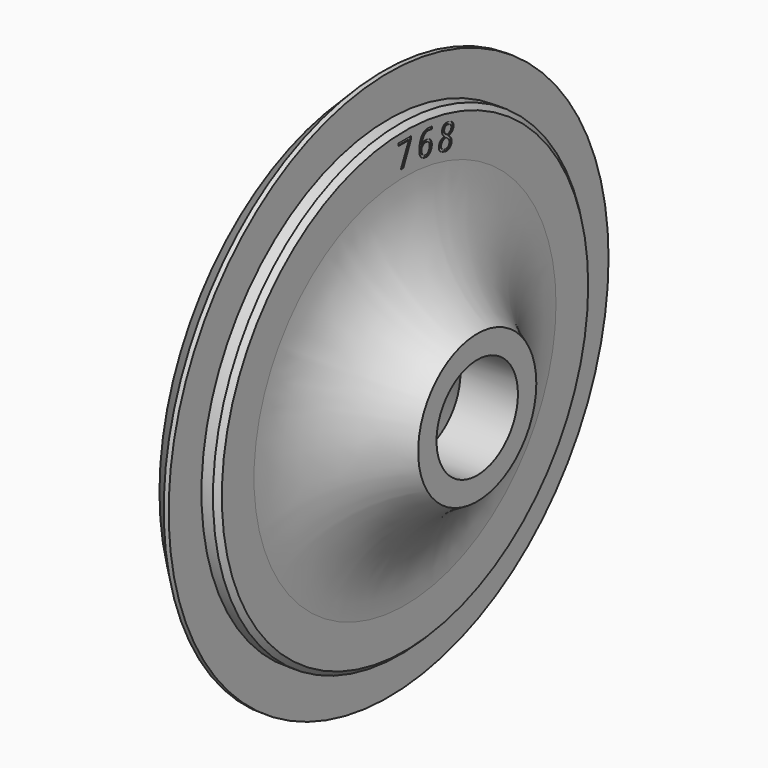
from build123d import *

# Parameters (mm, degrees)
F3_TEXT_SIZE = 2.0833333333
F4_DEPTH     = 0.05
F5_SIZE      = 0.3


# Not quite as in the source:
# - Text() gives the source's letters only with a copy of the font that has no kerning and outlines rounded to 1/6400 em; it was checked with that copy


with BuildPart() as f1:
    # F0 (on Top) → F1 (revolve)
    with BuildSketch(Plane.XY):
        with BuildLine():
            Line((-4.4, 11.5), (-4.4, 14.25))
            Line((-4.4, 14.25), (-5.4, 14.25))
            Line((-5.4, 14.25), (-5.4, 16.75))
            Line((-5.4, 16.75), (-5.7, 16.75))
            Line((-5.7, 16.75), (-7, 15.45))
            Line((-7, 15.45), (-7, 6))
            Line((-7, 6), (-6.4, 6))
            Line((-6.4, 6), (-3.5, 3.1))
            Line((-3.5, 3.1), (0, 3.1))
            Line((0, 3.1), (0, 4.5))
            ThreePointArc((0, 4.5), (-3.20864483, 7.3659946783), (-4.4, 11.5))
        make_face()
    revolve(axis=Axis((-3.5, 0, 0), (-1, 0, 0)))

    # F3 (on face) → F4 (cut)
    with BuildSketch(Plane.YZ.offset(-4.4)):
        with Locations((-0.6101888021, 12)):
            Text('7', F3_TEXT_SIZE, font='Open Sans', text_align=(TextAlign.LEFT, TextAlign.BOTTOM))
        with BuildLine():
            add(Edge.make_bspline(
                [(1.3911920227, 11.9124736168), (1.2492672408, 11.965505738), (1.168086207, 12.102022835)],
                knots=[0.2780169607, 0.2780169607, 0.2780169607, 1, 1, 1], degree=2))
            Line((1.3911920227, 11.9124736168), (1.5039988028, 11.9053764158))
            Line((1.5039988028, 11.9053764158), (1.6329910314, 11.8807698321))
            add(Edge.make_bspline(
                [(1.8658957751, 11.9728554781), (1.7668517571, 11.8921760098), (1.6329910314, 11.8807698321)],
                knots=[0, 0, 0, 0.6961452699, 0.6961452699, 0.6961452699], degree=2))
            add(Edge.make_bspline(
                [(2.0372600894, 12.3190162698), (2.0081707028, 12.0887500648), (1.8658957751, 11.9728554781)],
                knots=[0, 0, 0, 1, 1, 1], degree=2))
            add(Edge.make_bspline(
                [(1.9639386607, 12.6593399563), (2.063248784, 12.5247379706), (2.0372600894, 12.3190162698)],
                knots=[0, 0, 0, 1, 1, 1], degree=2))
            add(Edge.make_bspline(
                [(1.6656888708, 12.8190738665), (1.8646285374, 12.7939419421), (1.9639386607, 12.6593399563)],
                knots=[0, 0, 0, 1, 1, 1], degree=2))
            add(Edge.make_bspline(
                [(1.2923652787, 12.6897134657), (1.4254110915, 12.849428009), (1.6656888708, 12.8190738665)],
                knots=[0, 0, 0, 1, 1, 1], degree=2))
            Line((1.2923652787, 12.6897134657), (1.2804159806, 12.6912230132))
            add(Edge.make_bspline(
                [(1.4762395094, 13.1387963058), (1.332429483, 13.006854298), (1.2804159806, 12.6912230132)],
                knots=[0, 0, 0, 1, 1, 1], degree=2))
            add(Edge.make_bspline(
                [(1.8574207289, 13.2407513582), (1.6200495358, 13.2707383135), (1.4762395094, 13.1387963058)],
                knots=[0, 0, 0, 1, 1, 1], degree=2))
            add(Edge.make_bspline(
                [(2.0318631422, 13.1931217276), (1.9572135163, 13.2281445974), (1.8574207289, 13.2407513582)],
                knots=[0, 0, 0, 1, 1, 1], degree=2))
            Line((2.0318631422, 13.1931217276), (2.0501001068, 13.3374821676))
            add(Edge.make_bspline(
                [(1.8729447966, 13.3792204636), (1.9869475601, 13.3648185653), (2.0501001068, 13.3374821676)],
                knots=[0, 0, 0, 1, 1, 1], degree=2))
            add(Edge.make_bspline(
                [(1.3456378689, 13.2269867417), (1.5419169421, 13.4210390067), (1.8729447966, 13.3792204636)],
                knots=[0, 0, 0, 1, 1, 1], degree=2))
            add(Edge.make_bspline(
                [(1.0944031103, 12.5979154329), (1.1493587957, 13.0329344767), (1.3456378689, 13.2269867417)],
                knots=[0, 0, 0, 1, 1, 1], degree=2))
            add(Edge.make_bspline(
                [(1.168086207, 12.102022835), (1.0556444606, 12.2911091288), (1.0944031103, 12.5979154329)],
                knots=[0, 0, 0, 1, 1, 1], degree=2))
        make_face()
        with BuildLine():
            add(Edge.make_bspline(
                [(1.5255567916, 12.0266778564), (1.6689483695, 12.0085632875), (1.7594957026, 12.088994757)],
                knots=[0, 0, 0, 1, 1, 1], degree=2))
            add(Edge.make_bspline(
                [(1.3631201393, 12.100515938), (1.4306083143, 12.0386726385), (1.5255567916, 12.0266778564)],
                knots=[0, 0, 0, 1, 1, 1], degree=2))
            add(Edge.make_bspline(
                [(1.2666047187, 12.2572402731), (1.2956319644, 12.1623592375), (1.3631201393, 12.100515938)],
                knots=[0, 0, 0, 1, 1, 1], degree=2))
            add(Edge.make_bspline(
                [(1.2507146153, 12.456112498), (1.237577473, 12.3521213086), (1.2666047187, 12.2572402731)],
                knots=[0, 0, 0, 1, 1, 1], degree=2))
            add(Edge.make_bspline(
                [(1.3128222221, 12.5867280854), (1.259649504, 12.526839425), (1.2507146153, 12.456112498)],
                knots=[0, 0, 0, 1, 1, 1], degree=2))
            add(Edge.make_bspline(
                [(1.4464602893, 12.6745121437), (1.3659949402, 12.6466167459), (1.3128222221, 12.5867280854)],
                knots=[0, 0, 0, 1, 1, 1], degree=2))
            add(Edge.make_bspline(
                [(1.6176757137, 12.6909431409), (1.5269256385, 12.7024075415), (1.4464602893, 12.6745121437)],
                knots=[0, 0, 0, 1, 1, 1], degree=2))
            add(Edge.make_bspline(
                [(1.8270201595, 12.5793527447), (1.7639738776, 12.6724613848), (1.6176757137, 12.6909431409)],
                knots=[0, 0, 0, 1, 1, 1], degree=2))
            add(Edge.make_bspline(
                [(1.8715846852, 12.3399459407), (1.8900664413, 12.4862441047), (1.8270201595, 12.5793527447)],
                knots=[0, 0, 0, 1, 1, 1], degree=2))
            add(Edge.make_bspline(
                [(1.7594957026, 12.088994757), (1.8500430357, 12.1694262264), (1.8715846852, 12.3399459407)],
                knots=[0, 0, 0, 1, 1, 1], degree=2))
        make_face(mode=Mode.SUBTRACT)
        with BuildLine():
            Line((2.984278646, 11.6229979335), (3.1084826292, 11.582641613))
            add(Edge.make_bspline(
                [(3.3407163455, 11.6244062371), (3.239004536, 11.5744991717), (3.1084826292, 11.582641613)],
                knots=[0, 0, 0, 0.666283244, 0.666283244, 0.666283244], degree=2))
            add(Edge.make_bspline(
                [(3.5393535811, 11.8783969056), (3.4933718571, 11.6993099149), (3.3407163455, 11.6244062371)],
                knots=[0, 0, 0, 1, 1, 1], degree=2))
            add(Edge.make_bspline(
                [(3.5202228201, 12.1108345939), (3.5705207707, 11.9997850947), (3.5393535811, 11.8783969056)],
                knots=[0, 0, 0, 1, 1, 1], degree=2))
            add(Edge.make_bspline(
                [(3.3161551014, 12.3507625756), (3.4699248695, 12.2218840932), (3.5202228201, 12.1108345939)],
                knots=[0, 0, 0, 1, 1, 1], degree=2))
            add(Edge.make_bspline(
                [(3.568049378, 12.4561432869), (3.4796477929, 12.385410887), (3.3161551014, 12.3507625756)],
                knots=[0, 0, 0, 1, 1, 1], degree=2))
            add(Edge.make_bspline(
                [(3.683813327, 12.633445058), (3.6564509631, 12.5268756868), (3.568049378, 12.4561432869)],
                knots=[0, 0, 0, 1, 1, 1], degree=2))
            add(Edge.make_bspline(
                [(3.6335387466, 12.9160570829), (3.7252616415, 12.7948755848), (3.683813327, 12.633445058)],
                knots=[0, 0, 0, 1, 1, 1], degree=2))
            add(Edge.make_bspline(
                [(3.3447571031, 13.0878346681), (3.5418158517, 13.037238581), (3.6335387466, 12.9160570829)],
                knots=[0, 0, 0, 1, 1, 1], degree=2))
            add(Edge.make_bspline(
                [(3.0109417502, 13.0744004645), (3.1505360004, 13.1377021715), (3.3447571031, 13.0878346681)],
                knots=[0, 0, 0, 1, 1, 1], degree=2))
            add(Edge.make_bspline(
                [(2.8311134914, 12.8543976406), (2.8713474999, 13.0110987574), (3.0109417502, 13.0744004645)],
                knots=[0, 0, 0, 1, 1, 1], degree=2))
            add(Edge.make_bspline(
                [(2.838987399, 12.6396377139), (2.8027796827, 12.7440447413), (2.8311134914, 12.8543976406)],
                knots=[0, 0, 0, 1, 1, 1], degree=2))
            add(Edge.make_bspline(
                [(2.9914150698, 12.4237231833), (2.8751951154, 12.5352306864), (2.838987399, 12.6396377139)],
                knots=[0, 0, 0, 1, 1, 1], degree=2))
            add(Edge.make_bspline(
                [(2.5910685385, 12.1158256928), (2.6545362701, 12.363016187), (2.9914150698, 12.4237231833)],
                knots=[0, 0, 0, 1, 1, 1], degree=2))
            add(Edge.make_bspline(
                [(2.6417479014, 11.7974853225), (2.5434677398, 11.9304328221), (2.5910685385, 12.1158256928)],
                knots=[0, 0, 0, 1, 1, 1], degree=2))
            add(Edge.make_bspline(
                [(2.8349707002, 11.6514799475), (2.7081685053, 11.7076355191), (2.6417479014, 11.7974853225)],
                knots=[0.3241707912, 0.3241707912, 0.3241707912, 1, 1, 1], degree=2))
            Line((2.8349707002, 11.6514799475), (2.984278646, 11.6229979335))
        make_face()
        with BuildLine():
            add(Edge.make_bspline(
                [(2.7517619607, 12.0701976025), (2.7214043085, 11.9519623534), (2.7865785865, 11.8648198118)],
                knots=[0, 0, 0, 1, 1, 1], degree=2))
            add(Edge.make_bspline(
                [(2.864611575, 12.2361487897), (2.7791243246, 12.1767669738), (2.7517619607, 12.0701976025)],
                knots=[0, 0, 0, 1, 1, 1], degree=2))
            add(Edge.make_bspline(
                [(3.1132165763, 12.3208649627), (2.9500988255, 12.2955306057), (2.864611575, 12.2361487897)],
                knots=[0, 0, 0, 1, 1, 1], degree=2))
            add(Edge.make_bspline(
                [(3.3441396618, 12.1076496333), (3.2863130088, 12.2018117292), (3.1132165763, 12.3208649627)],
                knots=[0, 0, 0, 1, 1, 1], degree=2))
            add(Edge.make_bspline(
                [(3.3774373318, 11.9179534561), (3.4019663148, 12.0134875375), (3.3441396618, 12.1076496333)],
                knots=[0, 0, 0, 1, 1, 1], degree=2))
            add(Edge.make_bspline(
                [(3.2470462958, 11.7497845528), (3.3465939571, 11.797826443), (3.3774373318, 11.9179534561)],
                knots=[0, 0, 0, 1, 1, 1], degree=2))
            add(Edge.make_bspline(
                [(3.0005716315, 11.7394671052), (3.1474986344, 11.7017426627), (3.2470462958, 11.7497845528)],
                knots=[0, 0, 0, 1, 1, 1], degree=2))
            add(Edge.make_bspline(
                [(2.7865785865, 11.8648198118), (2.8517528645, 11.7776772701), (3.0005716315, 11.7394671052)],
                knots=[0, 0, 0, 1, 1, 1], degree=2))
        make_face(mode=Mode.SUBTRACT)
        with BuildLine():
            add(Edge.make_bspline(
                [(3.3087838148, 12.9555816174), (3.1855038617, 12.9872345295), (3.1003297681, 12.9460886351)],
                knots=[0, 0, 0, 1, 1, 1], degree=2))
            add(Edge.make_bspline(
                [(3.4903122269, 12.8464622774), (3.4339555319, 12.9234429829), (3.3087838148, 12.9555816174)],
                knots=[0, 0, 0, 1, 1, 1], degree=2))
            add(Edge.make_bspline(
                [(3.5210875403, 12.6698486686), (3.5466689219, 12.7694815719), (3.4903122269, 12.8464622774)],
                knots=[0, 0, 0, 1, 1, 1], degree=2))
            add(Edge.make_bspline(
                [(3.4217231258, 12.5263131832), (3.4978538171, 12.5793592912), (3.5210875403, 12.6698486686)],
                knots=[0, 0, 0, 1, 1, 1], degree=2))
            add(Edge.make_bspline(
                [(3.1895176683, 12.4504934191), (3.3455924345, 12.4732670752), (3.4217231258, 12.5263131832)],
                knots=[0, 0, 0, 1, 1, 1], degree=2))
            add(Edge.make_bspline(
                [(3.0080382263, 12.6357221665), (3.0494930217, 12.5556779911), (3.1895176683, 12.4504934191)],
                knots=[0, 0, 0, 1, 1, 1], degree=2))
            add(Edge.make_bspline(
                [(2.989817154, 12.8062557193), (2.9665834309, 12.7157663419), (3.0080382263, 12.6357221665)],
                knots=[0, 0, 0, 1, 1, 1], degree=2))
            add(Edge.make_bspline(
                [(3.1003297681, 12.9460886351), (3.0151556744, 12.9049427406), (2.989817154, 12.8062557193)],
                knots=[0, 0, 0, 1, 1, 1], degree=2))
        make_face(mode=Mode.SUBTRACT)
    extrude(amount=-F4_DEPTH, mode=Mode.SUBTRACT)

    # F5
    f5_edges = [f1.edges().sort_by_distance(p)[0] for p in [
        (-4.4, -14.25, 0),
    ]]
    chamfer(f5_edges, length=F5_SIZE)


solid = f1.part
